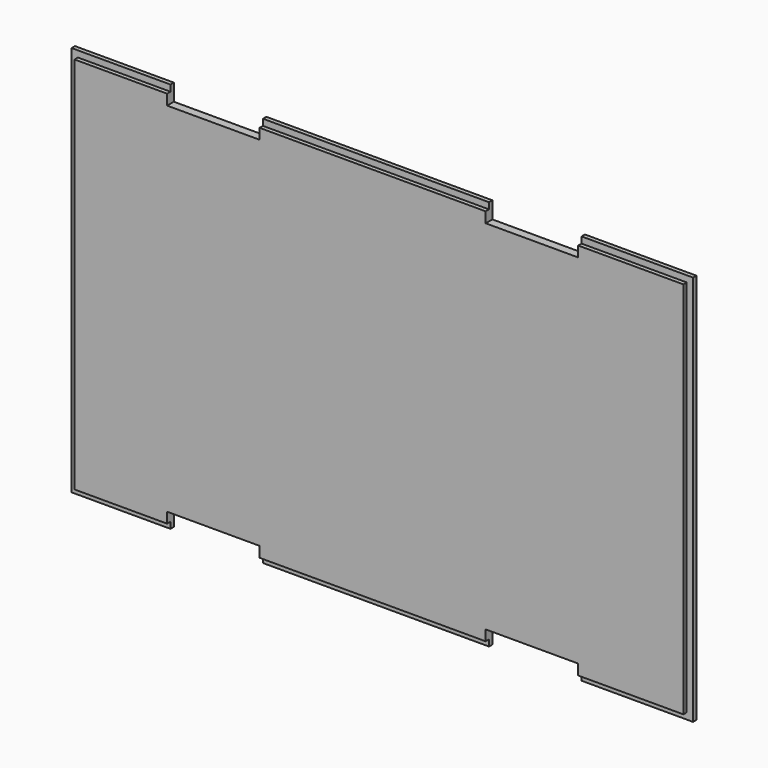
from build123d import *

# Parameters (mm, degrees)
F1_DEPTH      = 2.032
F0_W          = 54.61
F0_H          = 1.524
F2_DEPTH      = 1.016
F4_DEPTH      = 6.985
F5_DEPTH      = 5.461
F6_R          = 1.108982449
F7_DEPTH      = 25.4
F8_W          = 3.8512460887
F8_H          = 9.7791478038
F9_DEPTH      = 25.4
F10_T1_DEPTH  = 13.1787527424
F10_T3_DEPTH  = 8.89
F10_T5_DEPTH  = 10.16
F10_S9_W      = 2.54
F10_S9_H      = 2.54
F10_T10_DEPTH = 2.54
F10_S15_W     = 2.54
F10_S15_H     = 2.54
F10_T16_DEPTH = 2.54
F10_S21_W     = 2.54
F10_S21_H     = 2.54
F10_T22_DEPTH = 2.54
F10_S27_W     = 2.54
F10_S27_H     = 2.54
F10_T28_DEPTH = 2.54


# Not quite as in the source:
# - a fillet or chamfer that OpenCascade refuses, or shapes differently, is made with other operations: its cross-section is extruded or revolved along the edge and cut away or added


with BuildPart() as f1:
    # F0 (on Front) → F1 (new body)
    with BuildSketch(Plane.XZ):
        Polygon((-53.3597948303, 45.72), (-53.3597948303, 0), (93.7062051697, 0), (93.7062051697, 45.72), (68.3062051697, 45.72), (68.3062051697, 43.18), (45.9542051697, 43.18), (45.9542051697, 45.72), (-8.6557948303, 45.72), (-8.6557948303, 43.18), (-31.0077948303, 43.18), (-31.0077948303, 45.72), align=None)
        Polygon((93.7062051697, 0), (-53.3597948303, 0), (-53.3597948303, -45.72), (-31.0077948303, -45.72), (-31.0077948303, -43.18), (-8.6557948303, -43.18), (-8.6557948303, -45.72), (45.9542051697, -45.72), (45.9542051697, -43.18), (68.3062051697, -43.18), (68.3062051697, -45.72), (93.7062051697, -45.72), align=None)
    extrude(amount=F1_DEPTH)

    # F0 (on Front) → F2 (join)
    with BuildSketch(Plane.XZ):
        Polygon((-53.3597948303, -45.72), (-53.3597948303, 0), (-53.3597948303, 45.72), (-31.0077948303, 45.72), (-31.0077948303, 47.244), (-54.8837948303, 47.244), (-54.8837948303, 0), (-54.8837948303, -47.244), (-31.0077948303, -47.244), (-31.0077948303, -45.72), align=None)
        with Locations((18.6492051697, 46.482)):
            Rectangle(F0_W, F0_H)
        Polygon((93.7062051697, 45.72), (93.7062051697, 0), (93.7062051697, -45.72), (68.3062051697, -45.72), (68.3062051697, -47.244), (95.2302051697, -47.244), (95.2302051697, 12.7), (95.2302051697, 47.244), (68.3062051697, 47.244), (68.3062051697, 45.72), align=None)
        with Locations((18.6492051697, -46.482)):
            Rectangle(F0_W, F0_H)
    extrude(amount=F2_DEPTH)


with BuildPart() as f4:
    # F3 (on Top) → F4 (new body, symmetric)
    with BuildSketch(Plane.XY):
        with BuildLine():
            Line((-48.5492415086, 57.4260428548), (-50.5951202464, 57.4260428548))
            Line((-50.5951202464, 57.4260428548), (-50.5951202464, 48.0572901124))
            Line((-50.5951202464, 48.0572901124), (-35.3551202464, 48.0572901124))
            Line((-35.3551202464, 48.0572901124), (-35.3551202464, 57.4260428548))
            Line((-35.3551202464, 57.4260428548), (-37.4009989842, 57.4260428548))
            ThreePointArc((-37.4009989842, 57.4260428548), (-37.2004782482, 56.5618655999), (-37.1331202464, 55.6772901124))
            ThreePointArc((-37.1331202464, 55.6772901124), (-43.8596957339, 49.9026481143), (-48.5492415086, 57.4260428548))
        make_face()
        with BuildLine():
            Line((-37.4009989842, 57.4260428548), (-48.5492415086, 57.4260428548))
            ThreePointArc((-48.5492415086, 57.4260428548), (-43.8596957339, 49.9026481143), (-37.1331202464, 55.6772901124))
            ThreePointArc((-37.1331202464, 55.6772901124), (-37.2004782482, 56.5618655999), (-37.4009989842, 57.4260428548))
        make_face()
    extrude(amount=F4_DEPTH, both=True)

    # F3 (on Top) → F5 (cut, symmetric)
    with BuildSketch(Plane.XY):
        with BuildLine():
            Line((-37.4009989842, 57.4260428548), (-48.5492415086, 57.4260428548))
            ThreePointArc((-48.5492415086, 57.4260428548), (-43.8596957339, 49.9026481143), (-37.1331202464, 55.6772901124))
            ThreePointArc((-37.1331202464, 55.6772901124), (-37.2004782482, 56.5618655999), (-37.4009989842, 57.4260428548))
        make_face()
    extrude(amount=F5_DEPTH, both=True, mode=Mode.SUBTRACT)

    # F6 (on face) → F7 (cut)
    with BuildSketch(Plane.XY.offset(6.985)):
        with Locations((-43.0850237608, 53.2620474696)):
            Circle(F6_R)
    extrude(amount=-F7_DEPTH, mode=Mode.SUBTRACT)

    # F8 (on face) → F9 (cut)
    with BuildSketch(Plane.XZ.offset(-48.0572901124)):
        with Locations((-43.0246088654, -0.1216004603)):
            Rectangle(F8_W, F8_H)
    extrude(amount=-F9_DEPTH, mode=Mode.SUBTRACT)

    # F10: fillet of radius 2.54 on 8 edges, made by hand

    # F10_s2 → F10_t1 (cut)
    with BuildSketch(Plane.XZ.offset(-63.7760428548)):
        with BuildLine():
            ThreePointArc((-50.5951202464, 4.445), (-49.8511714706, 6.2410512242), (-48.0551202464, 6.985))
            Line((-48.0551202464, 6.985), (-50.5951202464, 6.985))
            Line((-50.5951202464, 6.985), (-50.5951202464, 4.445))
        make_face()
        with BuildLine():
            ThreePointArc((-50.5951202464, -4.445), (-49.8511714706, -6.2410512242), (-48.0551202464, -6.985))
            Line((-48.0551202464, -6.985), (-50.5951202464, -6.985))
            Line((-50.5951202464, -6.985), (-50.5951202464, -4.445))
        make_face()
        with BuildLine():
            ThreePointArc((-37.8951202464, 6.985), (-36.0990690222, 6.2410512242), (-35.3551202464, 4.445))
            Line((-35.3551202464, 4.445), (-35.3551202464, 6.985))
            Line((-35.3551202464, 6.985), (-37.8951202464, 6.985))
        make_face()
        with BuildLine():
            ThreePointArc((-37.8951202464, -6.985), (-36.0990690222, -6.2410512242), (-35.3551202464, -4.445))
            Line((-35.3551202464, -4.445), (-35.3551202464, -6.985))
            Line((-35.3551202464, -6.985), (-37.8951202464, -6.985))
        make_face()
    extrude(amount=F10_T1_DEPTH, mode=Mode.SUBTRACT)

    # F10_s4 → F10_t3 (cut)
    with BuildSketch(Plane.XY.offset(-4.445)):
        with BuildLine():
            ThreePointArc((-50.5951202464, 50.5972901124), (-49.8511714706, 48.8012388882), (-48.0551202464, 48.0572901124))
            Line((-48.0551202464, 48.0572901124), (-50.5951202464, 48.0572901124))
            Line((-50.5951202464, 48.0572901124), (-50.5951202464, 50.5972901124))
        make_face()
        with BuildLine():
            ThreePointArc((-37.8951202464, 48.0572901124), (-36.0990690222, 48.8012388882), (-35.3551202464, 50.5972901124))
            Line((-35.3551202464, 50.5972901124), (-35.3551202464, 48.0572901124))
            Line((-35.3551202464, 48.0572901124), (-37.8951202464, 48.0572901124))
        make_face()
    extrude(amount=F10_T3_DEPTH, mode=Mode.SUBTRACT)

    # F10_s6 → F10_t5 (cut)
    with BuildSketch(Plane.YZ.offset(-48.0551202464)):
        with BuildLine():
            ThreePointArc((50.5972901124, -6.985), (48.8012388882, -6.2410512242), (48.0572901124, -4.445))
            Line((48.0572901124, -4.445), (48.0572901124, -6.985))
            Line((48.0572901124, -6.985), (50.5972901124, -6.985))
        make_face()
        with BuildLine():
            ThreePointArc((48.0572901124, 4.445), (48.8012388882, 6.2410512242), (50.5972901124, 6.985))
            Line((50.5972901124, 6.985), (48.0572901124, 6.985))
            Line((48.0572901124, 6.985), (48.0572901124, 4.445))
        make_face()
    extrude(amount=F10_T5_DEPTH, mode=Mode.SUBTRACT)


with BuildPart() as f10_tool8:
    # F10_s9 → F10_t10 (new body)
    with BuildSketch(Plane.YZ.offset(-48.0551202464)):
        with Locations((49.3272901124, 5.715)):
            Rectangle(F10_S9_W, F10_S9_H)
    extrude(amount=-F10_T10_DEPTH)

    # F10_s11 → F10_t12 (revolve, cut)
    with BuildSketch(Plane(origin=(-48.0551202464, 50.5972901124, 4.445), x_dir=(0, 0.7071067812, -0.7071067812), z_dir=(0, 0.7071067812, 0.7071067812))):
        with BuildLine():
            ThreePointArc((0, -2.54), (2.54, 0), (0, 2.54))
            Line((0, 2.54), (0, -2.54))
        make_face()
    revolve(axis=Axis((-48.0551202464, 50.5972901124, 4.445), (-1, 0, 0)), mode=Mode.SUBTRACT)


with BuildPart() as f4_1:
    add(f4.part)

    # F10_t7: cut F10_tool8
    add(f10_tool8.part, mode=Mode.SUBTRACT)


with BuildPart() as f10_tool14:
    # F10_s15 → F10_t16 (new body)
    with BuildSketch(Plane.YZ.offset(-48.0551202464)):
        with Locations((49.3272901124, -5.715)):
            Rectangle(F10_S15_W, F10_S15_H)
    extrude(amount=-F10_T16_DEPTH)

    # F10_s17 → F10_t18 (revolve, cut)
    with BuildSketch(Plane(origin=(-48.0551202464, 50.5972901124, -4.445), x_dir=(0, 0.7071067812, 0.7071067812), z_dir=(0, -0.7071067812, 0.7071067812))):
        with BuildLine():
            ThreePointArc((0, -2.54), (2.54, 0), (0, 2.54))
            Line((0, 2.54), (0, -2.54))
        make_face()
    revolve(axis=Axis((-48.0551202464, 50.5972901124, -4.445), (-1, 0, 0)), mode=Mode.SUBTRACT)


with BuildPart() as f4_2:
    add(f4_1.part)

    # F10_t13: cut F10_tool14
    add(f10_tool14.part, mode=Mode.SUBTRACT)


with BuildPart() as f10_tool20:
    # F10_s21 → F10_t22 (new body)
    with BuildSketch(Plane.XZ.offset(-50.5972901124)):
        with Locations((-36.6251202464, 5.715)):
            Rectangle(F10_S21_W, F10_S21_H)
    extrude(amount=F10_T22_DEPTH)

    # F10_s23 → F10_t24 (revolve, cut)
    with BuildSketch(Plane(origin=(-37.8951202464, 50.5972901124, 4.445), x_dir=(-0.7071067812, 0, -0.7071067812), z_dir=(-0.7071067812, 0, 0.7071067812))):
        with BuildLine():
            ThreePointArc((0, -2.54), (2.54, 0), (0, 2.54))
            Line((0, 2.54), (0, -2.54))
        make_face()
    revolve(axis=Axis((-37.8951202464, 50.5972901124, 4.445), (0, -1, 0)), mode=Mode.SUBTRACT)


with BuildPart() as f4_3:
    add(f4_2.part)

    # F10_t19: cut F10_tool20
    add(f10_tool20.part, mode=Mode.SUBTRACT)


with BuildPart() as f10_tool26:
    # F10_s27 → F10_t28 (new body)
    with BuildSketch(Plane.XY.offset(-4.445)):
        with Locations((-36.6251202464, 49.3272901124)):
            Rectangle(F10_S27_W, F10_S27_H)
    extrude(amount=-F10_T28_DEPTH)

    # F10_s29 → F10_t30 (revolve, cut)
    with BuildSketch(Plane(origin=(-37.8951202464, 50.5972901124, -4.445), x_dir=(-0.7071067812, 0.7071067812, 0), z_dir=(-0.7071067812, -0.7071067812, 0))):
        with BuildLine():
            ThreePointArc((0, -2.54), (2.54, 0), (0, 2.54))
            Line((0, 2.54), (0, -2.54))
        make_face()
    revolve(axis=Axis((-37.8951202464, 50.5972901124, -4.445), (0, 0, -1)), mode=Mode.SUBTRACT)


with BuildPart() as f4_4:
    add(f4_3.part)

    # F10_t25: cut F10_tool26
    add(f10_tool26.part, mode=Mode.SUBTRACT)


solid = Compound([f1.part, f4_4.part])
